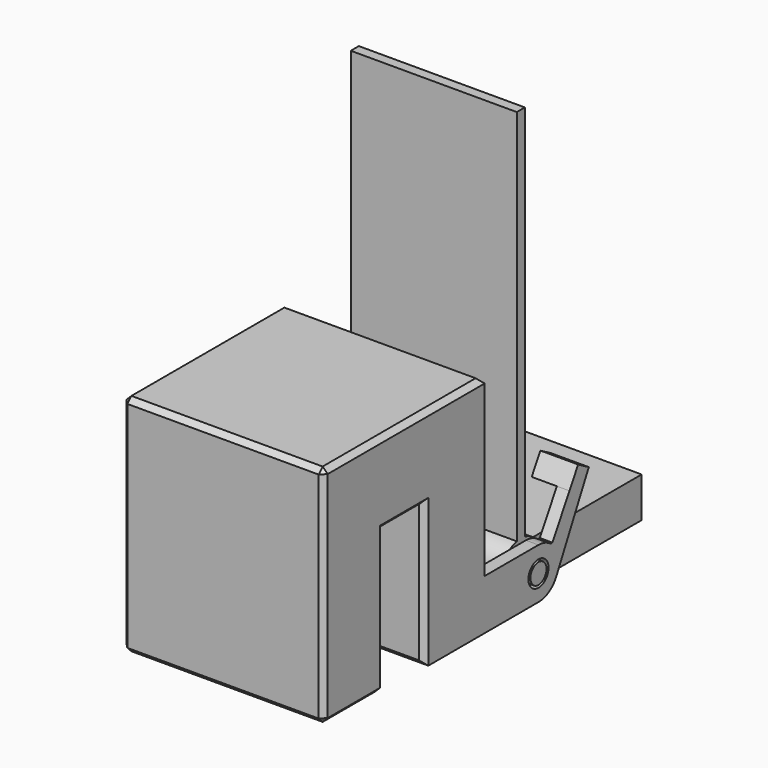
from build123d import *

# Parameters (mm, degrees)
F0_R     = 2.5
F1_DEPTH = 20
F2_DEPTH = 17.5
F0_R_2   = 2
F3_DEPTH = 16.5
F4_DEPTH = 20
F5_DEPTH = 12.5
F6_SIZE  = 1


# Not quite as in the source:
# - a feature names something its author has since deleted; it is built from what else it names


with BuildPart() as f1:
    # F0 (on Right) → F1 (new body, symmetric)
    with BuildSketch(Plane.YZ):
        with BuildLine():
            Line((-13.3660271764, -5), (0, -5))
            ThreePointArc((0, -5), (-4.974680765, -0.50254481), (-1, 4.8989794856))
            Line((-1, 4.8989794856), (-1, 5))
            Line((-1, 5), (-13.3660271764, 5))
            Line((-13.3660271764, 5), (-13.3660271764, -5))
        make_face()
        Polygon((-28.3660271764, -5), (-13.3660271764, -5), (-13.3660271764, 5), (-13.3660271764, 39.6839417517), (-53.3660271764, 39.6839417517), (-53.3660271764, 5), (-53.3660271764, -5), (-38.3660271764, -5), (-38.3660271764, 23.3722571284), (-28.3660271764, 23.3722571284), align=None)
        with BuildLine():
            ThreePointArc((-1, 4.8989794856), (-4.974680765, -0.50254481), (0, -5))
            ThreePointArc((0, -5), (1.5811388301, -4.7434164903), (3, -4))
            Line((3, -4), (3, 4))
            ThreePointArc((3, 4), (2.0498880528, 4.5604779323), (1, 4.8989794856))
            Line((1, 4.8989794856), (-1, 4.8989794856))
        make_face()
        Circle(F0_R, mode=Mode.SUBTRACT)
        with BuildLine():
            ThreePointArc((0, 5), (-0.50254481, 4.974680765), (-1, 4.8989794856))
            Line((-1, 4.8989794856), (1, 4.8989794856))
            ThreePointArc((1, 4.8989794856), (0.50254481, 4.974680765), (0, 5))
        make_face()
        with BuildLine():
            Line((-1, 5), (-1, 4.8989794856))
            ThreePointArc((-1, 4.8989794856), (-0.50254481, 4.974680765), (0, 5))
            Line((0, 5), (-1, 5))
        make_face()
        with BuildLine():
            Line((3, 4), (3, -4))
            ThreePointArc((3, -4), (3.8269094248, -3.2178819516), (4.4555102649, -2.2690148257))
            ThreePointArc((4.4555102649, -2.2690148257), (4.8619724045, -1.1667151914), (5, 0))
            ThreePointArc((5, 0), (4.5594723232, 2.0521238105), (3.3155151466, 3.7426406871))
            ThreePointArc((3.3155151466, 3.7426406871), (3.1603783548, 3.8745333467), (3, 4))
        make_face()
        Polygon((-28.3660271764, -5), (-13.3660271764, -5), (-13.3660271764, 5), (-13.3660271764, 39.6839417517), (-53.3660271764, 39.6839417517), (-53.3660271764, 5), (-53.3660271764, -5), (-38.3660271764, -5), (-38.3660271764, 23.3722571284), (-28.3660271764, 23.3722571284), align=None)
        with BuildLine():
            Line((3.4641016151, 4), (3, 4))
            ThreePointArc((3, 4), (3.1603783548, 3.8745333467), (3.3155151466, 3.7426406871))
            Line((3.3155151466, 3.7426406871), (3.4641016151, 4))
        make_face()
        with BuildLine():
            ThreePointArc((5, 0), (4.8619724045, -1.1667151914), (4.4555102649, -2.2690148257))
            Line((4.4555102649, -2.2690148257), (7.6480711023, 4))
            Line((7.6480711023, 4), (3.4641016151, 4))
            Line((3.4641016151, 4), (3.3155151466, 3.7426406871))
            ThreePointArc((3.3155151466, 3.7426406871), (4.5594723232, 2.0521238105), (5, 0))
        make_face()
        Polygon((7.6988384706, 11.3347793903), (11.6449917103, 11.8484814621), (12.5034797738, 13.5342361498), (9.8523915105, 15.0648426723), align=None)
        Polygon((3.4641016151, 4), (7.6480711023, 4), (11.6449917103, 11.8484814621), (7.6988384706, 11.3347793903), align=None)
    extrude(amount=F1_DEPTH, both=True)

    # F0 (on Right) → F2 (cut, symmetric)
    with BuildSketch(Plane.YZ):
        with BuildLine():
            Line((-13.3660271764, -5), (0, -5))
            ThreePointArc((0, -5), (-4.974680765, -0.50254481), (-1, 4.8989794856))
            Line((-1, 4.8989794856), (-1, 5))
            Line((-1, 5), (-13.3660271764, 5))
            Line((-13.3660271764, 5), (-13.3660271764, -5))
        make_face()
        with BuildLine():
            ThreePointArc((-1, 4.8989794856), (-4.974680765, -0.50254481), (0, -5))
            ThreePointArc((0, -5), (1.5811388301, -4.7434164903), (3, -4))
            Line((3, -4), (3, 4))
            ThreePointArc((3, 4), (2.0498880528, 4.5604779323), (1, 4.8989794856))
            Line((1, 4.8989794856), (-1, 4.8989794856))
        make_face()
        Circle(F0_R, mode=Mode.SUBTRACT)
        with BuildLine():
            Line((-1, 5), (-1, 4.8989794856))
            ThreePointArc((-1, 4.8989794856), (-0.50254481, 4.974680765), (0, 5))
            Line((0, 5), (-1, 5))
        make_face()
        with BuildLine():
            ThreePointArc((0, 5), (-0.50254481, 4.974680765), (-1, 4.8989794856))
            Line((-1, 4.8989794856), (1, 4.8989794856))
            ThreePointArc((1, 4.8989794856), (0.50254481, 4.974680765), (0, 5))
        make_face()
        with BuildLine():
            Line((3, 4), (3, -4))
            ThreePointArc((3, -4), (3.8269094248, -3.2178819516), (4.4555102649, -2.2690148257))
            ThreePointArc((4.4555102649, -2.2690148257), (4.8619724045, -1.1667151914), (5, 0))
            ThreePointArc((5, 0), (4.5594723232, 2.0521238105), (3.3155151466, 3.7426406871))
            ThreePointArc((3.3155151466, 3.7426406871), (3.1603783548, 3.8745333467), (3, 4))
        make_face()
        Polygon((3.4641016151, 4), (7.6480711023, 4), (11.6449917103, 11.8484814621), (7.6988384706, 11.3347793903), align=None)
        with BuildLine():
            ThreePointArc((5, 0), (4.8619724045, -1.1667151914), (4.4555102649, -2.2690148257))
            Line((4.4555102649, -2.2690148257), (7.6480711023, 4))
            Line((7.6480711023, 4), (3.4641016151, 4))
            Line((3.4641016151, 4), (3.3155151466, 3.7426406871))
            ThreePointArc((3.3155151466, 3.7426406871), (4.5594723232, 2.0521238105), (5, 0))
        make_face()
        with BuildLine():
            Line((3.4641016151, 4), (3, 4))
            ThreePointArc((3, 4), (3.1603783548, 3.8745333467), (3.3155151466, 3.7426406871))
            Line((3.3155151466, 3.7426406871), (3.4641016151, 4))
        make_face()
    extrude(amount=F2_DEPTH, both=True, mode=Mode.SUBTRACT)

    # F0 (on Right) → F5 (cut, symmetric)
    with BuildSketch(Plane.YZ):
        Polygon((7.6988384706, 11.3347793903), (11.6449917103, 11.8484814621), (12.5034797738, 13.5342361498), (9.8523915105, 15.0648426723), align=None)
    extrude(amount=F5_DEPTH, both=True, mode=Mode.SUBTRACT)

    # F6
    f6_edges = [f1.edges().sort_by_distance(p)[0] for p in [
        (0, -53.366027, 39.683942),
        (20, -33.366027, 39.683942),
        (0, -13.366027, 39.683942),
        (-20, -33.366027, 39.683942),
        (20, -53.366027, 17.341971),
        (20, -45.866027, -5),
        (0, -38.366027, -5),
        (0, -28.366027, -5),
        (20, -38.366027, 9.186129),
        (20, -33.366027, 23.372257),
        (20, -28.366027, 9.186129),
        (0, -53.366027, -5),
        (-20, -45.866027, -5),
        (-20, -53.366027, 17.341971),
    ]]
    chamfer(f6_edges, length=F6_SIZE)


with BuildPart() as f3:
    # F0 (on Right) → F3 (new body, symmetric)
    with BuildSketch(Plane.YZ):
        with BuildLine():
            Line((-1, 5), (0, 5))
            ThreePointArc((0, 5), (0.50254481, 4.974680765), (1, 4.8989794856))
            Line((1, 4.8989794856), (1, 80))
            Line((1, 80), (-1, 80))
            Line((-1, 80), (-1, 5))
        make_face()
        with BuildLine():
            Line((-1, 5), (-1, 4.8989794856))
            ThreePointArc((-1, 4.8989794856), (-0.50254481, 4.974680765), (0, 5))
            Line((0, 5), (-1, 5))
        make_face()
        with BuildLine():
            ThreePointArc((0, 5), (-0.50254481, 4.974680765), (-1, 4.8989794856))
            Line((-1, 4.8989794856), (1, 4.8989794856))
            ThreePointArc((1, 4.8989794856), (0.50254481, 4.974680765), (0, 5))
        make_face()
        with BuildLine():
            ThreePointArc((-1, 4.8989794856), (-4.974680765, -0.50254481), (0, -5))
            ThreePointArc((0, -5), (1.5811388301, -4.7434164903), (3, -4))
            Line((3, -4), (3, 4))
            ThreePointArc((3, 4), (2.0498880528, 4.5604779323), (1, 4.8989794856))
            Line((1, 4.8989794856), (-1, 4.8989794856))
        make_face()
        Circle(F0_R, mode=Mode.SUBTRACT)
        with BuildLine():
            Line((3, 4), (3, -4))
            ThreePointArc((3, -4), (3.8269094248, -3.2178819516), (4.4555102649, -2.2690148257))
            ThreePointArc((4.4555102649, -2.2690148257), (4.8619724045, -1.1667151914), (5, 0))
            ThreePointArc((5, 0), (4.5594723232, 2.0521238105), (3.3155151466, 3.7426406871))
            ThreePointArc((3.3155151466, 3.7426406871), (3.1603783548, 3.8745333467), (3, 4))
        make_face()
        Circle(F0_R)
        Circle(F0_R_2, mode=Mode.SUBTRACT)
        Circle(F0_R_2)
        with BuildLine():
            ThreePointArc((4.4555102649, -2.2690148257), (3.8269094248, -3.2178819516), (3, -4))
            Line((3, -4), (30, -4))
            Line((30, -4), (30, 4))
            Line((30, 4), (7.6480711023, 4))
            Line((7.6480711023, 4), (4.4555102649, -2.2690148257))
        make_face()
        with BuildLine():
            ThreePointArc((5, 0), (4.8619724045, -1.1667151914), (4.4555102649, -2.2690148257))
            Line((4.4555102649, -2.2690148257), (7.6480711023, 4))
            Line((7.6480711023, 4), (3.4641016151, 4))
            Line((3.4641016151, 4), (3.3155151466, 3.7426406871))
            ThreePointArc((3.3155151466, 3.7426406871), (4.5594723232, 2.0521238105), (5, 0))
        make_face()
        with BuildLine():
            Line((3.4641016151, 4), (3, 4))
            ThreePointArc((3, 4), (3.1603783548, 3.8745333467), (3.3155151466, 3.7426406871))
            Line((3.3155151466, 3.7426406871), (3.4641016151, 4))
        make_face()
    extrude(amount=F3_DEPTH, both=True)

    # F0 (on Right) → F4 (join, symmetric)
    with BuildSketch(Plane.YZ):
        Circle(F0_R_2)
    extrude(amount=F4_DEPTH, both=True)


solid = Compound([f1.part, f3.part])
